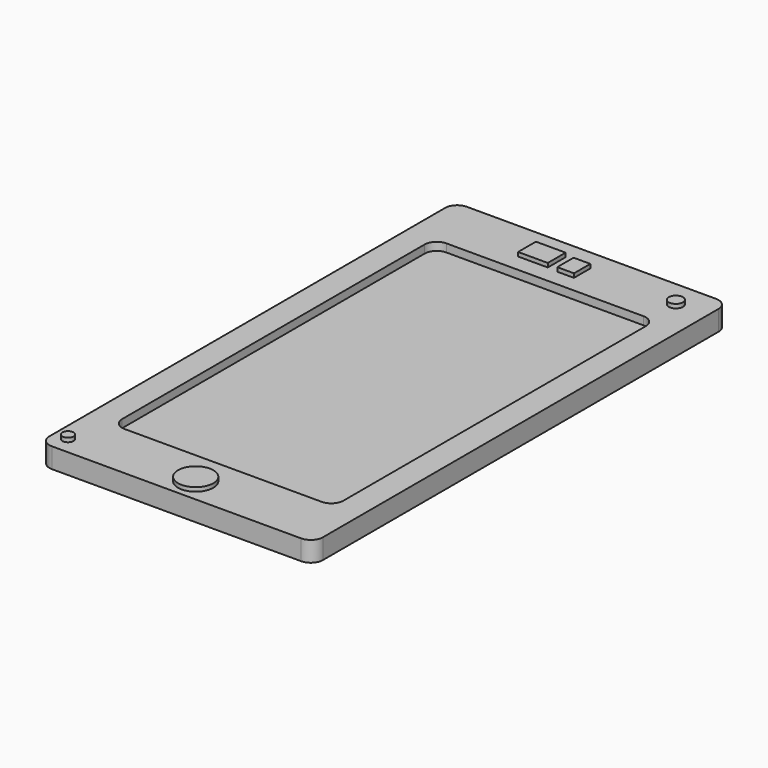
from build123d import *

# Parameters (mm, degrees)
F1_W      = 68
F1_H      = 129
F1_W_2    = 55
F1_H_2    = 100
F2_DEPTH  = 5
F3_R      = 3
F4_R      = 3
F5_W      = 55
F5_H      = 100
F6_DEPTH  = 3
F0_R      = 4.3933448382
F7_DEPTH  = 6
F8_W      = 4.1563683189
F8_H      = 5.0799995661
F9_DEPTH  = 6
F10_W     = 7.3890909553
F10_H     = 5.5418238044
F11_DEPTH = 6
F12_R     = 1.7585544961
F13_DEPTH = 6
F24_R     = 1.3854540884
F25_DEPTH = 6


# Not quite as in the source:
# - the program builds the solid bodies; features that only make, move or delete a surface that nothing else refers to are left out


with BuildPart() as f2:
    # F1 (on Top) → F2 (new body)
    with BuildSketch(Plane.XY):
        Rectangle(F1_W, F1_H)
        Rectangle(F1_W_2, F1_H_2, mode=Mode.SUBTRACT)
    extrude(amount=F2_DEPTH)

    # F3
    f3_edges = [f2.edges().sort_by_distance(p)[0] for p in [
        (-34, 64.5, 2.5),
        (34, 64.5, 2.5),
        (34, -64.5, 2.5),
        (-34, -64.5, 2.5),
    ]]
    fillet(f3_edges, radius=F3_R)

    # F4
    f4_edges = [f2.edges().sort_by_distance(p)[0] for p in [
        (-27.5, 50, 2.5),
        (27.5, 50, 2.5),
        (-27.5, -50, 2.5),
        (27.5, -50, 2.5),
    ]]
    fillet(f4_edges, radius=F4_R)

    # F5 (on Top) → F6 (join)
    with BuildSketch(Plane.XY):
        Rectangle(F5_W, F5_H)
    extrude(amount=F6_DEPTH)

    # F0 (on Top) → F7 (join)
    with BuildSketch(Plane.XY):
        with Locations((0, -58.5363544524)):
            Circle(F0_R)
    extrude(amount=F7_DEPTH)

    # F8 (on Top) → F9 (join)
    with BuildSketch(Plane.XY):
        with Locations((1.8472720403, 56.6872768104)):
            Rectangle(F8_W, F8_H)
    extrude(amount=F9_DEPTH)

    # F10 (on Top) → F11 (join)
    with BuildSketch(Plane.XY):
        with Locations((-6.4654545859, 57.1491010487)):
            Rectangle(F10_W, F10_H)
    extrude(amount=F11_DEPTH)

    # F12 (on Top) → F13 (join)
    with BuildSketch(Plane.XY):
        with Locations((26.3236332685, 57.8418262303)):
            Circle(F12_R)
    extrude(amount=F13_DEPTH)

    # F24 (on Top) → F25 (join)
    with BuildSketch(Plane.XY):
        with Locations((-30.4799992591, -60.15272066)):
            Circle(F24_R)
    extrude(amount=F25_DEPTH)


solid = f2.part
